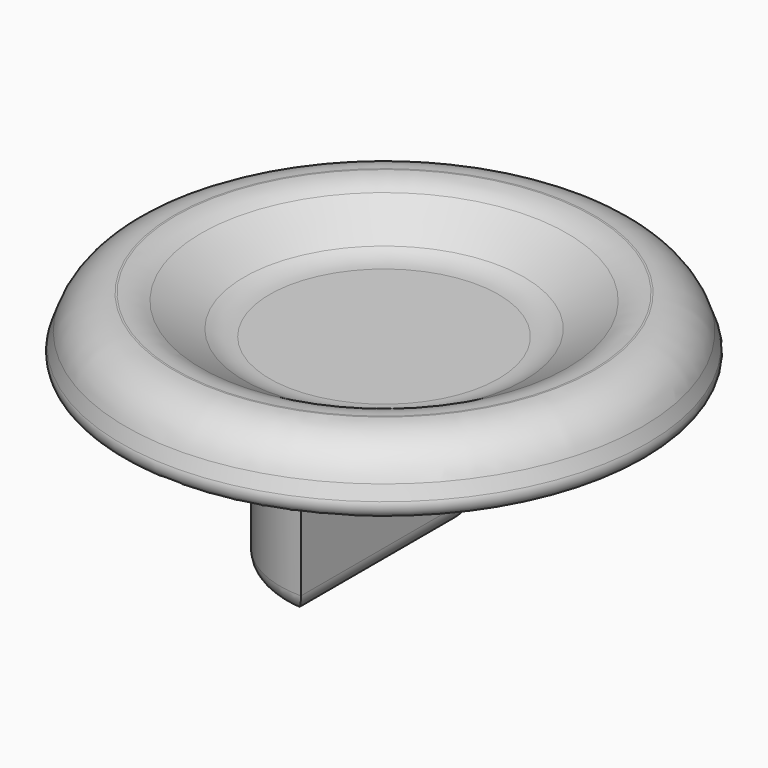
from build123d import *

# Parameters (mm, degrees)
F2_W     = 4.05
F2_H     = 8.1
F3_DEPTH = 6
F4_R     = 0.75
F5_R     = 2
F6_R     = 0.5


with BuildPart() as f1:
    # F0 (on Front) → F1 (revolve)
    with BuildSketch(Plane.XZ):
        Polygon((4.05, 0), (4.05, 6), (5.5, 7), (10.5, 7), (9.5900744143, 9.5), (7.5900744143, 9.5), (4.991998203, 8), (0, 8), (0, 0), align=None)
    revolve(axis=Axis((0, 0, 4), (0, 0, -1)))

    # F2 (on face) → F3 (cut)
    with BuildSketch(Plane(origin=(0, 0, 0), x_dir=(1, 0, 0), z_dir=(0, 0, -1))):
        with Locations((2.025, 0)):
            Rectangle(F2_W, F2_H)
    extrude(amount=-F3_DEPTH, mode=Mode.SUBTRACT)

    # F4
    f4_edges = [f1.edges().sort_by_distance(p)[0] for p in [
        (0, 0, 0),
        (0, 0, 6),
        (-4.05, 0, 0),
    ]]
    fillet(f4_edges, radius=F4_R)

    # F5
    f5_edges = [f1.edges().sort_by_distance(p)[0] for p in [
        (-9.590074, 0, 9.5),
        (-7.590074, 0, 9.5),
        (-4.991998, 0, 8),
    ]]
    fillet(f5_edges, radius=F5_R)

    # F6
    f6_edges = [f1.edges().sort_by_distance(p)[0] for p in [
        (-10.5, 0, 7),
    ]]
    fillet(f6_edges, radius=F6_R)


solid = f1.part
